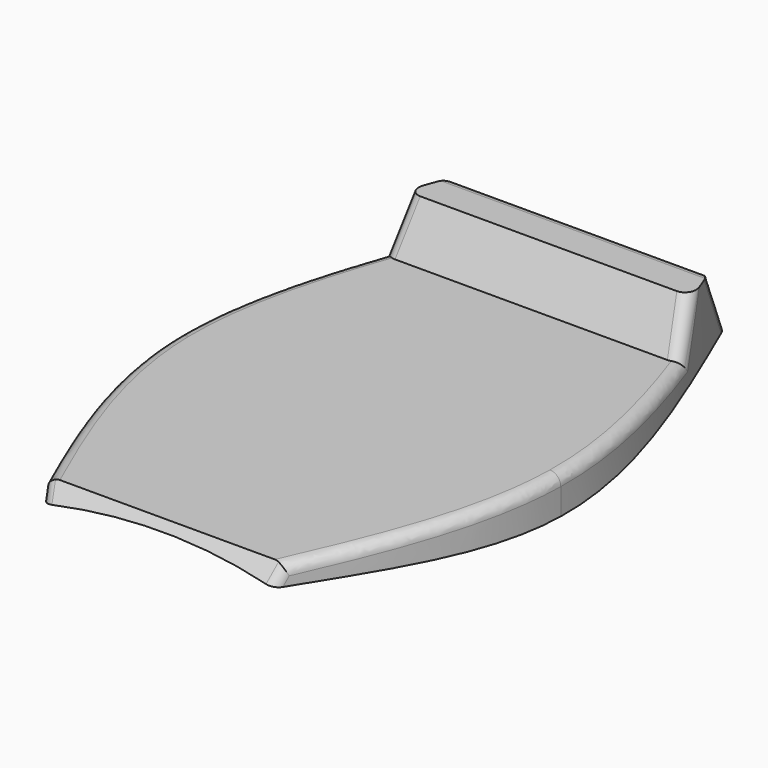
from build123d import *

# Parameters (mm, degrees)
F2_DEPTH = 10.0393754
F0_W     = 162.54427284
F0_H     = 91.0251736641
F3_DEPTH = 36.576
F4_R     = 1.27
F6_DEPTH = 57.15


# Not quite as in the source:
# - a feature names something its author has since deleted; it is built from what else it names


with BuildPart() as f2:
    # F1 (on Top) → F2 (new body)
    with BuildSketch(Plane.XY):
        with BuildLine():
            Line((22.098, 1.000200763), (0, 1.000200763))
            Line((0, 1.000200763), (0, -9.4128639907))
            Line((0, -9.4128639907), (0, -30.5107254535))
            Line((0, -30.5107254535), (12.7, -30.5107254535))
            add(Edge.make_bspline(
                [(22.098, 1.000200763), (21.9117681537, -9.8773063583), (17.3058840768, -20.1940159059), (12.7, -30.5107254535)],
                knots=[0.5153173826, 0.5153173826, 0.5153173826, 0.5153173826, 1, 1, 1, 1], degree=3))
        make_face()
        with BuildLine():
            Line((0, 36.9631461799), (0, 11.4132655167))
            Line((0, 11.4132655167), (0, 1.000200763))
            Line((0, 1.000200763), (22.098, 1.000200763))
            add(Edge.make_bspline(
                [(12.7, 36.9631461799), (17.498001392, 24.7641879428), (22.296002784, 12.5652297057), (22.098, 1.000200763)],
                knots=[0, 0, 0, 0, 0.5153173826, 0.5153173826, 0.5153173826, 0.5153173826], degree=3))
            Line((12.7, 36.9631461799), (0, 36.9631461799))
        make_face()
        with BuildLine():
            Line((0, 1.000200763), (0, 11.4132655167))
            Line((0, 11.4132655167), (0, 36.9631461799))
            Line((0, 36.9631461799), (-12.7, 36.9631461799))
            add(Edge.make_bspline(
                [(-12.7, 36.9631461799), (-17.498001392, 24.7641879428), (-22.296002784, 12.5652297057), (-22.098, 1.000200763)],
                knots=[0, 0, 0, 0, 0.5153173826, 0.5153173826, 0.5153173826, 0.5153173826], degree=3))
            Line((-22.098, 1.000200763), (0, 1.000200763))
        make_face()
        with BuildLine():
            Line((0, -9.4128639907), (0, 1.000200763))
            Line((0, 1.000200763), (-22.098, 1.000200763))
            add(Edge.make_bspline(
                [(-22.098, 1.000200763), (-21.9117681537, -9.8773063583), (-17.3058840768, -20.1940159059), (-12.7, -30.5107254535)],
                knots=[0.5153173826, 0.5153173826, 0.5153173826, 0.5153173826, 1, 1, 1, 1], degree=3))
            Line((-12.7, -30.5107254535), (0, -30.5107254535))
            Line((0, -30.5107254535), (0, -9.4128639907))
        make_face()
    extrude(amount=F2_DEPTH)

    # F0 (on Right) → F3 (cut, symmetric)
    with BuildSketch(Plane.YZ):
        with Locations((14.1260512173, 4.4935680926)):
            Rectangle(F0_W, F0_H)
        Polygon((3.2016009947, 0), (-30.665065672, 0), (-28.0743391016, 4.3514131215), (-17.965065672, 4.3514131215), (3.2016009947, 4.3514131215), (24.3682676614, 4.3514131215), (26.8577352928, 10.0393698853), (31.0910686261, 10.0393698853), (37.0682676614, 0), align=None, mode=Mode.SUBTRACT)
    extrude(amount=F3_DEPTH, both=True, mode=Mode.SUBTRACT)

    # F4
    f4_edges = [f2.edges().sort_by_distance(p)[0] for p in [
        (-21.914013, -2.246239, 4.351413),
        (-17.021737, 25.613292, 7.196056),
        (17.021737, 25.613292, 7.196056),
        (21.914013, -2.246239, 4.351413),
        (-13.852046, 34.027829, 5.106754),
        (13.852046, 34.027829, 5.106754),
        (0, 31.091069, 10.03937),
        (13.243552, -29.292588, 2.305229),
        (-13.243552, -29.292588, 2.305229),
    ]]
    fillet(f4_edges, radius=F4_R)

    # F5 (on Front) → F6 (cut, symmetric)
    with BuildSketch(Plane.XZ):
        with BuildLine():
            Line((22.8318180889, -5.8896035279), (22.8318180889, -0.1746035279))
            ThreePointArc((22.8318180889, -0.1746035279), (-0.0372941666, 3.3380936757), (-22.9064058512, -0.1746072442))
            Line((-22.9064058512, -0.1746072442), (-22.9064058512, -5.8896072442))
            Line((-22.9064058512, -5.8896072442), (22.8318180889, -5.8896035279))
        make_face()
        with BuildLine():
            Line((22.8318180889, -11.6046035279), (22.8318180889, -5.8896035279))
            Line((22.8318180889, -5.8896035279), (-22.9064058512, -5.8896072442))
            Line((-22.9064058512, -5.8896072442), (-22.9064058512, -11.6046072442))
            ThreePointArc((-22.9064058512, -11.6046072442), (-0.0372941666, -8.0919063243), (22.8318180889, -11.6046035279))
        make_face()
    extrude(amount=F6_DEPTH, both=True, mode=Mode.SUBTRACT)


solid = f2.part
